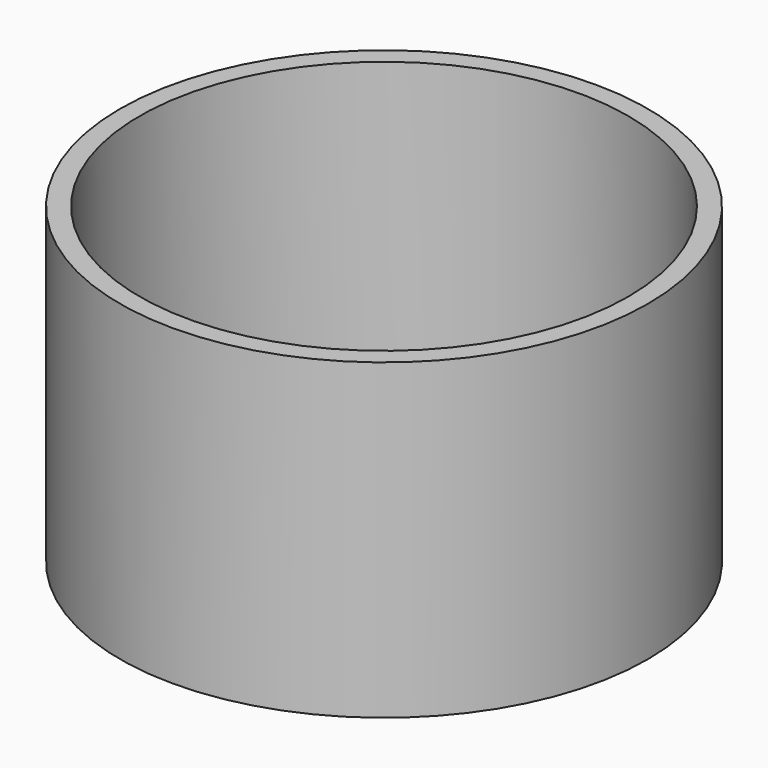
from build123d import *

# Parameters (mm, degrees)
F1_R         = 13.5
F2_DEPTH     = 16
F0_R         = 12.5
F3_DEPTH     = 15
F5_R         = 2.9
F6_DEPTH     = 25.4
F7_TEXT_SIZE = 4.4056421353
F8_DEPTH     = 1


# Not quite as in the source:
# - Text() gives the source's letters only with a copy of the font that has no kerning and outlines rounded to 1/6400 em; it was checked with that copy


with BuildPart() as f2:
    # F1 (on Top) → F2 (new body)
    with BuildSketch(Plane.XY):
        Circle(F1_R)
    extrude(amount=-F2_DEPTH)

    # F0 (on Top) → F3 (cut)
    with BuildSketch(Plane.XY):
        Circle(F0_R)
    extrude(amount=-F3_DEPTH, mode=Mode.SUBTRACT)

    # F5 (on offset) → F6 (cut)
    with BuildSketch(Plane.XY.offset(-16)):
        Circle(F5_R)
    extrude(amount=F6_DEPTH, mode=Mode.SUBTRACT)

    # F7 (on face) → F8 (join)
    with BuildSketch(Plane(origin=(0, 0, -16), x_dir=(1, 0, 0), z_dir=(0, 0, -1))):
        with Locations((-9.0399105102, 4.114203155)):
            Text('Amman', F7_TEXT_SIZE, font='Open Sans', text_align=(TextAlign.LEFT, TextAlign.BOTTOM))
    extrude(amount=F8_DEPTH)


solid = f2.part
